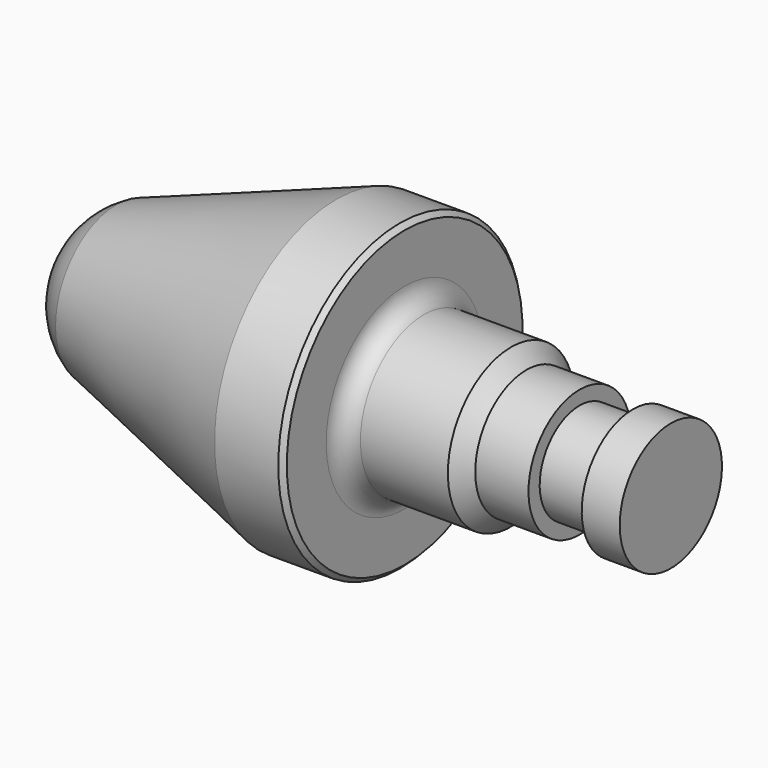
from build123d import *

# Parameters (mm, degrees)
F2_SIZE = 0.396875


# Not quite as in the source:
# - a feature names something its author has since deleted; it is built from what else it names


with BuildPart() as f1:
    # F0 (on Front) → F1 (revolve)
    with BuildSketch(Plane.XZ):
        with BuildLine():
            Line((0, 8.1915), (0, 12.7))
            Line((0, 12.7), (-5.715, 12.7))
            Line((-5.715, 12.7), (-24.0689650903, 6.35))
            ThreePointArc((-24.0689650903, 6.35), (-26.8959476355, 3.7184476355), (-27.94, 0))
            Line((-27.94, 0), (22.225, 0))
            Line((22.225, 0), (22.225, 5.334))
            Line((22.225, 5.334), (19.05, 5.334))
            Line((19.05, 5.334), (19.05, 4.1656))
            Line((19.05, 4.1656), (14.605, 4.1656))
            Line((14.605, 4.1656), (14.605, 5.334))
            Line((14.605, 5.334), (10.16, 5.334))
            Line((10.16, 5.334), (8.89, 6.604))
            Line((8.89, 6.604), (1.5875, 6.604))
            ThreePointArc((1.5875, 6.604), (0.4649679849, 7.0689679849), (0, 8.1915))
        make_face()
    revolve(axis=Axis((-2.8575, 0, 0), (-1, 0, 0)))

    # F2
    f2_edges = [f1.edges().sort_by_distance(p)[0] for p in [
        (0, 0, -12.7),
    ]]
    chamfer(f2_edges, length=F2_SIZE)


solid = f1.part
